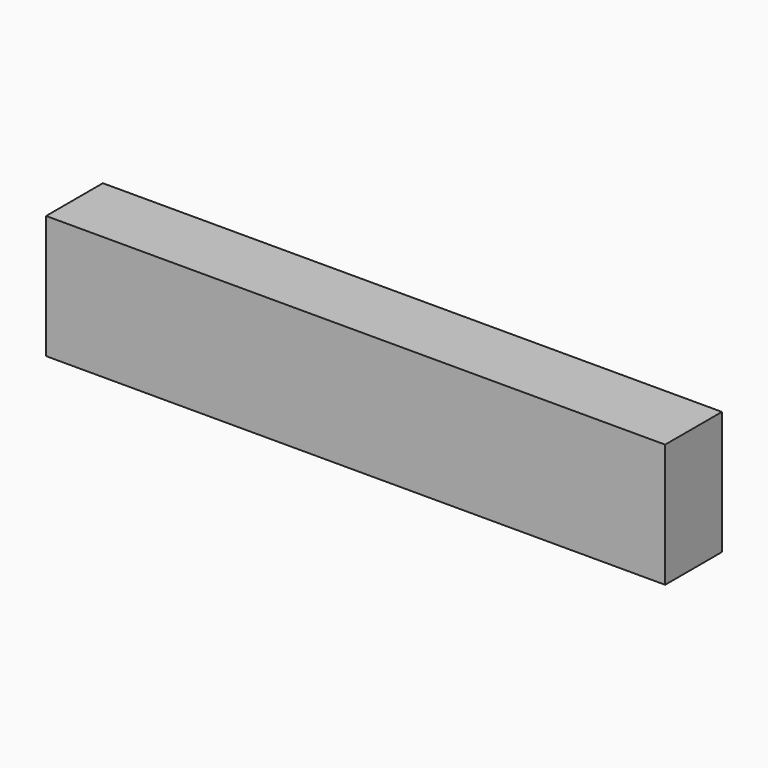
from build123d import *

# Parameters (mm, degrees)
F0_W     = 60.157597065
F0_H     = 193.3636292815
F1_DEPTH = 25.4
F2_W     = 95.6334322691
F2_H     = 193.3636292815
F3_DEPTH = 346.1655080318
F4_W     = 36.0463038087
F4_H     = 45.3125461936
F4_H_2   = 28.3587574959
F4_H_3   = 42.0287176967
F4_H_4   = 40.5834168196
F5_DEPTH = 25.4
F6_W     = 173.7615093589
F6_H     = 156.2834382057
F7_DEPTH = 25.4
F8_W     = 111.7356568575
F8_H     = 18.2048454881
F8_W_2   = 24.7079984665
F8_H_2   = 0.1422166824
F8_H_3   = 10.7772573829
F8_W_3   = 37.4475419521
F9_DEPTH = 3015.5396461487


with BuildPart() as f1:
    # F0 (on Front) → F1 (new body)
    with BuildSketch(Plane.XZ):
        Polygon((0, -95.5383777618), (0, 0), (0, 97.8252515197), (-34.4947949052, 97.8252515197), (-34.4947949052, -95.5383777618), align=None)
        Polygon((-34.4947949052, 97.8252515197), (0, 97.8252515197), (16.5538433939, 97.8252515197), (16.5538433939, 130.5804550648), (-34.4947949052, 130.5804550648), (-34.4947949052, 120.8282783628), align=None)
        Polygon((16.5538433939, -95.5383777618), (0, -95.5383777618), (-34.4947949052, -95.5383777618), (-34.4947949052, -108.2416400313), (16.5538433939, -108.2416400313), (16.5538433939, -98.9981219172), align=None)
        Polygon((95.6334322691, 97.8252515197), (95.6334322691, 0), (95.6334322691, -95.5383777618), (16.5538433939, -95.5383777618), (16.5538433939, -98.9981219172), (149.6599912643, -98.9981219172), (149.6599912643, 130.5804550648), (16.5538433939, 130.5804550648), (16.5538433939, 97.8252515197), align=None)
        with Locations((-64.5735934377, 1.1434368789)):
            Rectangle(F0_W, F0_H)
        Polygon((-94.6523919702, 97.8252515197), (-34.4947949052, 97.8252515197), (-34.4947949052, 120.8282783628), (-151.3080298901, 120.8282783628), (-151.3080298901, -95.5383777618), (-94.6523919702, -95.5383777618), align=None)
    extrude(amount=F1_DEPTH)

    # F2 (on face) → F3 (join)
    with BuildSketch(Plane(origin=(0, 0, 0), x_dir=(-1, 0, 0), z_dir=(0, 1, 0))):
        Polygon((151.3080298901, 108.881868422), (-95.6334322691, 108.881868422), (-95.6334322691, 97.8252515197), (0, 97.8252515197), (0, -95.5383777618), (-95.6334322691, -95.5383777618), (-95.6334322691, -98.9981219172), (-16.5538433939, -98.9981219172), (-16.5538433939, -108.2416400313), (34.4947949052, -108.2416400313), (34.4947949052, -95.5383777618), (151.3080298901, -95.5383777618), align=None)
        with Locations((-47.8167161345, 1.1434368789)):
            Rectangle(F2_W, F2_H)
    extrude(amount=-F3_DEPTH)

    # F4 (on face) → F5 (join)
    with BuildSketch(Plane(origin=(0, 0, 0), x_dir=(-1, 0, 0), z_dir=(0, 1, 0))):
        Polygon((78.8774639368, 89.2047658563), (-77.3589983582, 89.2047658563), (-77.3589983582, 43.8922196627), (-77.3589983582, 15.5334621668), (-77.3589983582, -26.4952555299), (-77.3589983582, -67.0786723495), (78.8774639368, -67.0786723495), align=None)
        with Locations((-95.3821502626, 66.5484927595)):
            Rectangle(F4_W, F4_H)
        with Locations((-95.3821502626, 29.7128409147)):
            Rectangle(F4_W, F4_H_2)
        with Locations((-95.3821502626, -5.4808966815)):
            Rectangle(F4_W, F4_H_3)
        with Locations((-95.3821502626, -46.7869639397)):
            Rectangle(F4_W, F4_H_4)
    extrude(amount=F5_DEPTH)

    # F6 (on face) → F7 (join)
    with BuildSketch(Plane(origin=(0, 25.4, 0), x_dir=(-1, 0, 0), z_dir=(0, 1, 0))):
        with Locations((-8.0032907426, 11.0630467534)):
            Rectangle(F6_W, F6_H)
    extrude(amount=F7_DEPTH)

    # F8 (on face) → F9 (intersect)
    with BuildSketch(Plane.YZ.offset(94.8840454221)):
        Polygon((50.8, 89.2047658563), (50.8, -67.0786723495), (74.874997139, -67.0786723495), (186.6106539965, -67.0786723495), (186.6106539965, 89.3469825387), (112.9555404186, 89.3469825387), (112.9555404186, 70.3727975488), (75.5079984665, 70.3727975488), (75.5079984665, 89.2047658563), align=None)
        with Locations((130.7428255677, -76.1810950935)):
            Rectangle(F8_W, F8_H)
        Polygon((-6.2784720212, 89.2047658563), (50.8, 89.2047658563), (50.8, 89.3469825387), (50.8, 100.1242399216), (-6.2784720212, 100.1242399216), align=None)
        with Locations((63.1539992332, 89.2758741975)):
            Rectangle(F8_W_2, F8_H_2)
        with Locations((63.1539992332, 94.7356112301)):
            Rectangle(F8_W_2, F8_H_3)
        Polygon((75.5079984665, 89.3469825387), (75.5079984665, 89.2047658563), (75.5079984665, 70.3727975488), (112.9555404186, 70.3727975488), (112.9555404186, 89.3469825387), align=None)
        with Locations((94.2317694426, 94.7356112301)):
            Rectangle(F8_W_3, F8_H_3)
    extrude(amount=F9_DEPTH, mode=Mode.INTERSECT)


solid = f1.part
